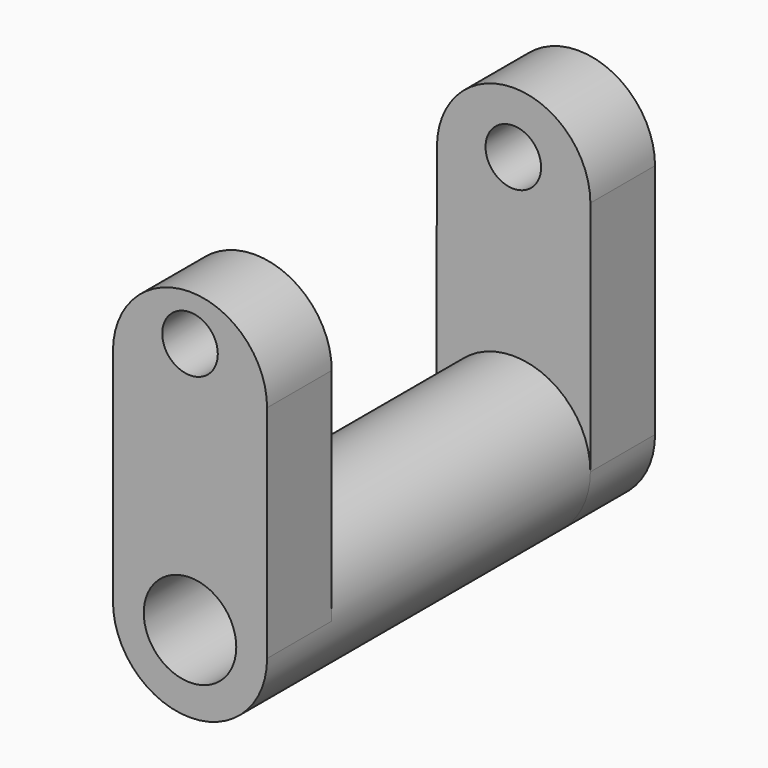
from build123d import *

# Parameters (mm, degrees)
F0_R     = 24.2146085631
F1_DEPTH = 101.6
F3_DEPTH = 25.4
F5_DEPTH = 25.4
F6_R     = 8.7323577449
F6_R_2   = 14.5344701606
F7_DEPTH = 254


with BuildPart() as f1:
    # F0 (on Front) → F1 (new body)
    with BuildSketch(Plane.XZ):
        Circle(F0_R)
    extrude(amount=F1_DEPTH)

    # F2 (on face) → F3 (join)
    with BuildSketch(Plane.XZ.offset(101.6)):
        with BuildLine():
            Line((-24.2146085631, 69.3517327309), (-24.2146085631, 0))
            ThreePointArc((-24.2146085631, 0), (0, 24.2146085631), (24.2146085631, 0))
            Line((24.2146085631, 0), (24.2146085631, 69.3517327309))
            ThreePointArc((24.2146085631, 69.3517327309), (0, 93.5663412939), (-24.2146085631, 69.3517327309))
        make_face()
        with BuildLine():
            ThreePointArc((24.2146085631, 0), (0, 24.2146085631), (-24.2146085631, 0))
            ThreePointArc((-24.2146085631, 0), (0, -24.2146085631), (24.2146085631, 0))
        make_face()
    extrude(amount=F3_DEPTH)

    # F4 (on face) → F5 (join)
    with BuildSketch(Plane(origin=(0, 0, 0), x_dir=(-1, 0, 0), z_dir=(0, 1, 0))):
        with BuildLine():
            ThreePointArc((23.9994246513, 74.3728801608), (-0.1075919559, 98.4102157735), (-24.2146085631, 74.3728801608))
            Line((-24.2146085631, 74.3728801608), (23.9994246513, 74.3728801608))
        make_face()
        with BuildLine():
            Line((-24.2146085631, 74.3728801608), (-24.2146085631, 0))
            ThreePointArc((-24.2146085631, 0), (-0.0350465649, 24.2145832011), (24.2145071151, 0.0700930563))
            Line((24.2145071151, 0.0700930563), (23.9994246513, 74.3728801608))
            Line((23.9994246513, 74.3728801608), (-24.2146085631, 74.3728801608))
        make_face()
        with BuildLine():
            ThreePointArc((24.2145071151, 0.0700930563), (-0.0350465649, 24.2145832011), (-24.2146085631, 0))
            ThreePointArc((-24.2146085631, 0), (0, -24.2146085631), (24.2146085631, 0))
            ThreePointArc((24.2146085631, 0), (24.2145832011, 0.0350465649), (24.2145071151, 0.0700930563))
        make_face()
    extrude(amount=F5_DEPTH)

    # F6 (on face) → F7 (cut)
    with BuildSketch(Plane.XZ.offset(127)):
        with Locations((0, 79.1887566447)):
            Circle(F6_R)
        Circle(F6_R_2)
    extrude(amount=-F7_DEPTH, mode=Mode.SUBTRACT)


solid = f1.part
